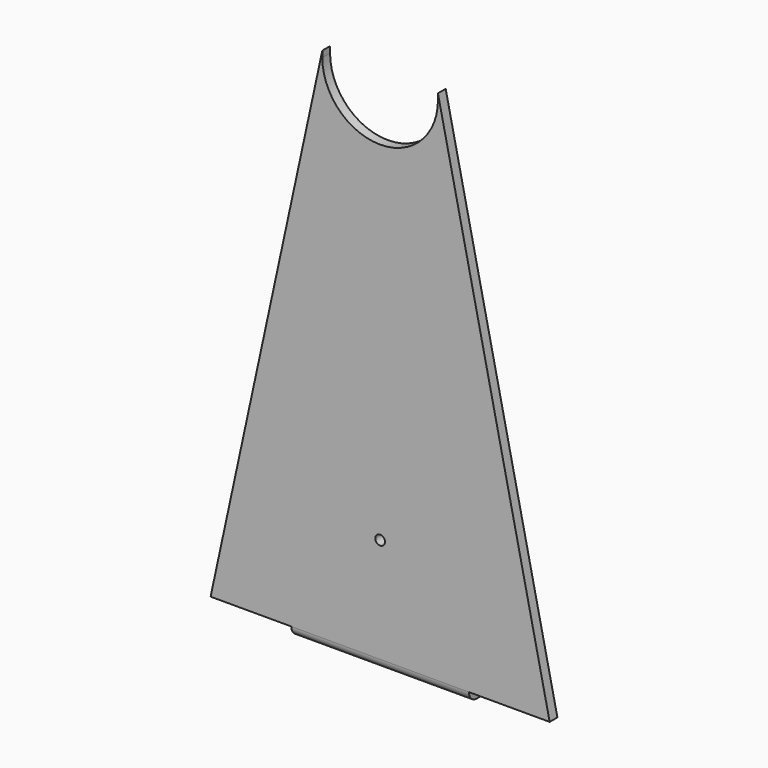
from build123d import *

# Parameters (mm, degrees)
F0_R     = 1.5
F1_DEPTH = 3
F2_W     = 55
F2_H     = 3
F3_DEPTH = 25
F4_R     = 3
F5_R     = 3
F6_DEPTH = 163.1321276775


with BuildPart() as f1:
    # F0 (on Front) → F1 (new body)
    with BuildSketch(Plane.XZ):
        with BuildLine():
            Line((454.8277321524, 574.7700988736), (454.8277321524, 576.6820907487))
            Line((454.8277321524, 576.6820907487), (420.231500864, 416.5509630712))
            Line((420.231500864, 416.5509630712), (495.9500458773, 416.5509630712))
            Line((495.9500458773, 416.5509630712), (525.231500864, 416.5509630712))
            Line((525.231500864, 416.5509630712), (490.6352695757, 576.6820907487))
            Line((490.6352695757, 576.6820907487), (490.6352695757, 574.7700988736))
            ThreePointArc((490.6352695757, 574.7700988736), (472.731500864, 556.866330162), (454.8277321524, 574.7700988736))
        make_face()
        with Locations((472.731500864, 449.0509630712)):
            Circle(F0_R, mode=Mode.SUBTRACT)
    extrude(amount=F1_DEPTH)

    # F2 (on face) → F3 (join)
    with BuildSketch(Plane.XZ.offset(3)):
        with Locations((472.731500864, 415.0509630712)):
            Rectangle(F2_W, F2_H)
    extrude(amount=-F3_DEPTH)

    # F4
    f4_edges = [f1.edges().sort_by_distance(p)[0] for p in [
        (472.731501, -3, 413.550963),
        (472.731501, 0, 416.550963),
    ]]
    fillet(f4_edges, radius=F4_R)

    # F5 (on face) → F6 (cut, through all)
    with BuildSketch(Plane(origin=(0, 0, 413.5509630712), x_dir=(1, 0, 0), z_dir=(0, 0, -1))):
        with Locations((472.731500864, -6.5)):
            Circle(F5_R)
    extrude(amount=-F6_DEPTH, mode=Mode.SUBTRACT)


solid = f1.part
